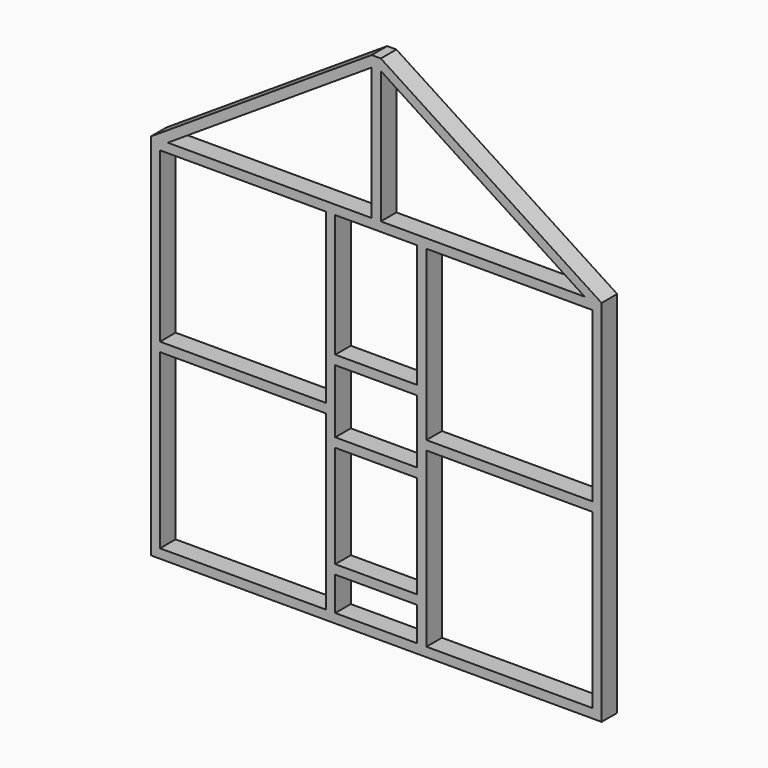
from build123d import *

# Parameters (mm, degrees)
F0_W     = 810
F0_H     = 45
F0_W_2   = 400
F1_DEPTH = 95


# Not quite as in the source:
# - a feature names something its author has since deleted; it is built from what else it names


with BuildPart() as f1:
    # F0 (on Front) → F1 (new body)
    with BuildSketch(Plane.XZ):
        Polygon((1100, -628.1681121112), (1100, -583.1681121112), (1055, -583.1681121112), (245, -583.1681121112), (200, -583.1681121112), (-200, -583.1681121112), (-245, -583.1681121112), (-1055, -583.1681121112), (-1100, -583.1681121112), (-1100, -628.1681121112), align=None)
        Polygon((1055, -583.1681121112), (1100, -583.1681121112), (1100, 1126.8318878888), (1055, 1126.8318878888), (1055, 304.8318878888), (1055, 259.8318878888), align=None)
        Polygon((1055, 1126.8318878888), (1100, 1126.8318878888), (1100, 1171.8318878888), (1017.398329114, 1171.8318878888), (22.5, 1171.8318878888), (-22.5, 1171.8318878888), (-1017.398329114, 1171.8318878888), (-1100, 1171.8318878888), (-1100, 1126.8318878888), (-1055, 1126.8318878888), (-245, 1126.8318878888), (-200, 1126.8318878888), (200, 1126.8318878888), (245, 1126.8318878888), align=None)
        Polygon((1017.398329114, 1171.8318878888), (1100, 1171.8318878888), (22.5, 1871.8318878888), (22.5, 1818.1695494942), align=None)
        Polygon((-1100, 1126.8318878888), (-1100, -583.1681121112), (-1055, -583.1681121112), (-1055, 259.8318878888), (-1055, 304.8318878888), (-1055, 1126.8318878888), align=None)
        Polygon((22.5, 1818.1695494942), (22.5, 1871.8318878888), (-22.5, 1871.8318878888), (-22.5, 1818.1695494942), (-22.5, 1171.8318878888), (22.5, 1171.8318878888), align=None)
        Polygon((-22.5, 1818.1695494942), (-22.5, 1871.8318878888), (-1100, 1171.8318878888), (-1017.398329114, 1171.8318878888), align=None)
        Polygon((-245, -583.1681121112), (-200, -583.1681121112), (-200, -418.1681121112), (-200, -373.1681121112), (-200, 126.8318878888), (-200, 171.8318878888), (-200, 481.8318878888), (-200, 526.8318878888), (-200, 1126.8318878888), (-245, 1126.8318878888), (-245, 304.8318878888), (-245, 259.8318878888), align=None)
        Polygon((200, -583.1681121112), (245, -583.1681121112), (245, 259.8318878888), (245, 304.8318878888), (245, 1126.8318878888), (200, 1126.8318878888), (200, 526.8318878888), (200, 481.8318878888), (200, 171.8318878888), (200, 126.8318878888), (200, -373.1681121112), (200, -418.1681121112), align=None)
        with Locations((-650, 282.3318878888)):
            Rectangle(F0_W, F0_H)
        with Locations((0, -395.6681121112)):
            Rectangle(F0_W_2, F0_H)
        with Locations((0, 149.3318878888)):
            Rectangle(F0_W_2, F0_H)
        with Locations((650, 282.3318878888)):
            Rectangle(F0_W, F0_H)
        with Locations((0, 504.3318878888)):
            Rectangle(F0_W_2, F0_H)
    extrude(amount=F1_DEPTH)


solid = f1.part
